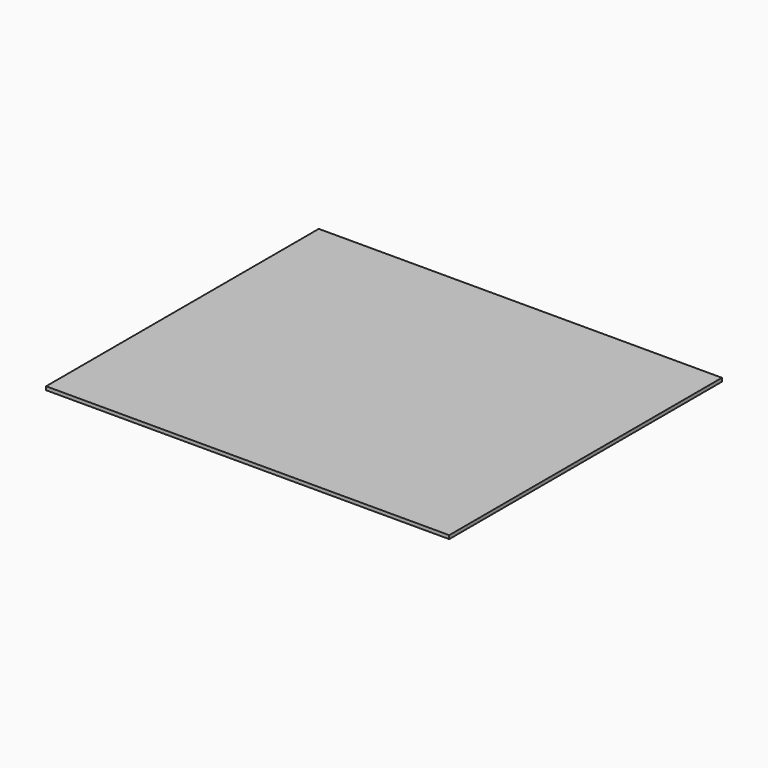
from build123d import *

# Parameters (mm, degrees)
F0_W     = 546.1
F0_H     = 461.772
F1_DEPTH = 4.7625


# Not quite as in the source:
# - a length typed as a fraction of an inch, garbled in the dataset ("3 / 203.2 mm" for 3/8 in), is restored


with BuildPart() as f1:
    # F0 (on Top) → F1 (new body)
    with BuildSketch(Plane.XY):
        with Locations((-21.4692822933, 63.4286133127)):
            Rectangle(F0_W, F0_H)
    extrude(amount=-F1_DEPTH)


solid = f1.part
